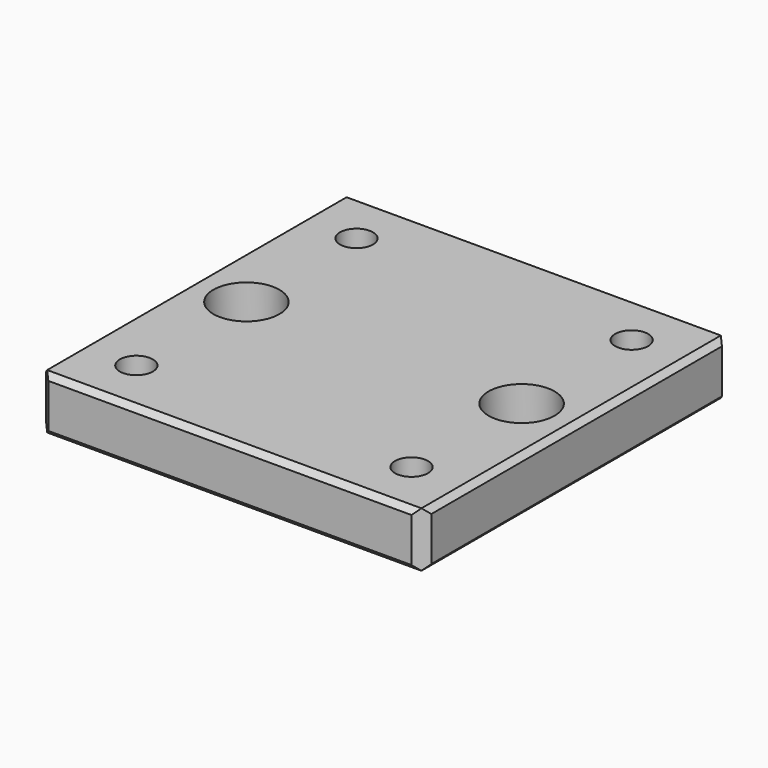
from build123d import *

# Parameters (mm, degrees)
F0_W     = 35
F0_H     = 35
F0_R     = 1.5
F0_R_2   = 2
F1_DEPTH = 5
F2_R     = 3
F3_DEPTH = 3.5
F4_SIZE  = 1
F5_SIZE  = 0.49999


# Not quite as in the source:
# - a fillet or chamfer is up to 0.001 mm smaller than in the source, because OpenCascade refuses the exact size


with BuildPart() as f1:
    # F0 (on Top) → F1 (new body)
    with BuildSketch(Plane.XY):
        Rectangle(F0_W, F0_H)
        with Locations((-12.5, -12.5)):
            Circle(F0_R, mode=Mode.SUBTRACT)
        with Locations((12.5, -12.5)):
            Circle(F0_R, mode=Mode.SUBTRACT)
        with Locations((-12.5, 0)):
            Circle(F0_R_2, mode=Mode.SUBTRACT)
        with Locations((-12.5, 12.5)):
            Circle(F0_R, mode=Mode.SUBTRACT)
        with Locations((12.5, 0)):
            Circle(F0_R_2, mode=Mode.SUBTRACT)
        with Locations((12.5, 12.5)):
            Circle(F0_R, mode=Mode.SUBTRACT)
    extrude(amount=F1_DEPTH)

    # F2 (on face) → F3 (cut)
    with BuildSketch(Plane.XY.offset(5)):
        with Locations((-12.5, 0)):
            Circle(F2_R)
        with Locations((12.5, 0)):
            Circle(F2_R)
    extrude(amount=-F3_DEPTH, mode=Mode.SUBTRACT)

    # F4
    f4_edges = [f1.edges().sort_by_distance(p)[0] for p in [
        (-17.5, -17.5, 2.5),
        (-17.5, 17.5, 2.5),
        (17.5, -17.5, 2.5),
        (17.5, 17.5, 2.5),
    ]]
    chamfer(f4_edges, length=F4_SIZE)

    # F5 (size 0.5 in the source; OpenCascade refuses exactly that, so slightly less here)
    f5_edges = [f1.edges().sort_by_distance(p)[0] for p in [
        (17.5, 0, 5),
        (0, 17.5, 5),
        (-17.5, 0, 5),
        (17.5, 0, 0),
        (0, -17.5, 5),
        (0, -17.5, 0),
        (0, 17.5, 0),
        (-17.5, 0, 0),
    ]]
    chamfer(f5_edges, length=F5_SIZE)


solid = f1.part
